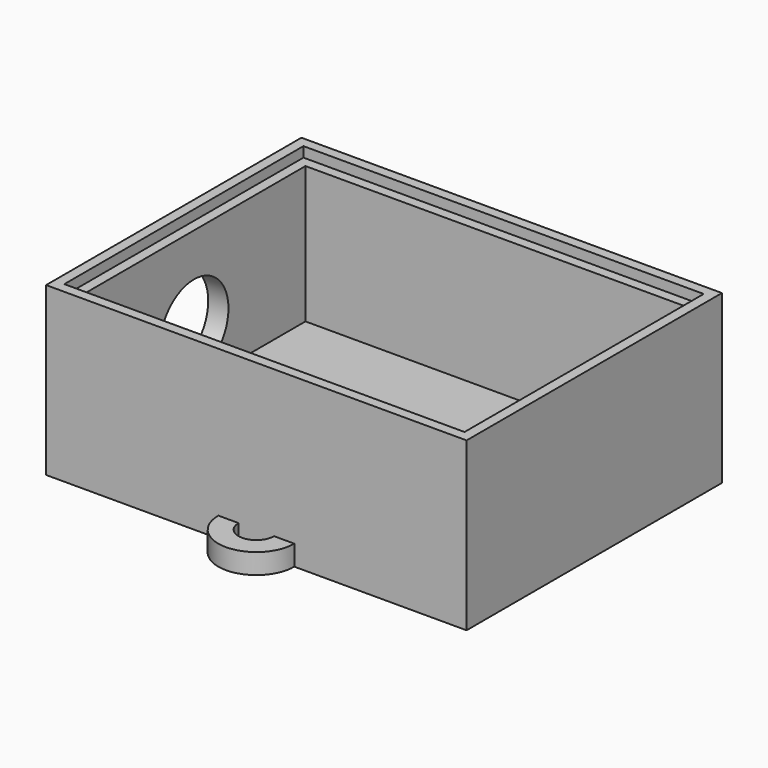
from build123d import *

# Parameters (mm, degrees)
F0_W     = 79
F0_H     = 59
F0_W_2   = 75
F0_H_2   = 55
F1_DEPTH = 4
F2_DEPTH = 31
F3_DEPTH = 33
F4_R     = 8.5
F5_DEPTH = 41.501


# Not quite as in the source:
# - a feature names something its author has since deleted; it is built from what else it names


with BuildPart() as f1:
    # F0 (on Top) → F1 (new body)
    with BuildSketch(Plane.XY):
        Polygon((41.5, -31.5), (41.5, 31.5), (7.5, 31.5), (3.5, 31.5), (-3.5, 31.5), (-7.5, 31.5), (-41.5, 31.5), (-41.5, -31.5), (-7.5, -31.5), (-3.5, -31.5), (3.5, -31.5), (7.5, -31.5), align=None)
        Rectangle(F0_W, F0_H, mode=Mode.SUBTRACT)
        Rectangle(F0_W, F0_H)
        Rectangle(F0_W_2, F0_H_2, mode=Mode.SUBTRACT)
        Rectangle(F0_W_2, F0_H_2)
        with BuildLine():
            ThreePointArc((-7.5, -31.5), (0, -39), (7.5, -31.5))
            Line((7.5, -31.5), (3.5, -31.5))
            ThreePointArc((3.5, -31.5), (0, -35), (-3.5, -31.5))
            Line((-3.5, -31.5), (-7.5, -31.5))
        make_face()
        with BuildLine():
            Line((3.5, 31.5), (7.5, 31.5))
            ThreePointArc((7.5, 31.5), (0, 39), (-7.5, 31.5))
            Line((-7.5, 31.5), (-3.5, 31.5))
            ThreePointArc((-3.5, 31.5), (0, 35), (3.5, 31.5))
        make_face()
    extrude(amount=F1_DEPTH)

    # F0 (on Top) → F2 (join)
    with BuildSketch(Plane.XY):
        Rectangle(F0_W, F0_H)
        Rectangle(F0_W_2, F0_H_2, mode=Mode.SUBTRACT)
    extrude(amount=F2_DEPTH)

    # F0 (on Top) → F3 (join)
    with BuildSketch(Plane.XY):
        Polygon((41.5, -31.5), (41.5, 31.5), (7.5, 31.5), (3.5, 31.5), (-3.5, 31.5), (-7.5, 31.5), (-41.5, 31.5), (-41.5, -31.5), (-7.5, -31.5), (-3.5, -31.5), (3.5, -31.5), (7.5, -31.5), align=None)
        Rectangle(F0_W, F0_H, mode=Mode.SUBTRACT)
    extrude(amount=F3_DEPTH)

    # F4 (on Right) → F5 (cut, through all)
    with BuildSketch(Plane.YZ):
        with Locations((0, 14)):
            Circle(F4_R)
    extrude(amount=-F5_DEPTH, mode=Mode.SUBTRACT)


solid = f1.part
